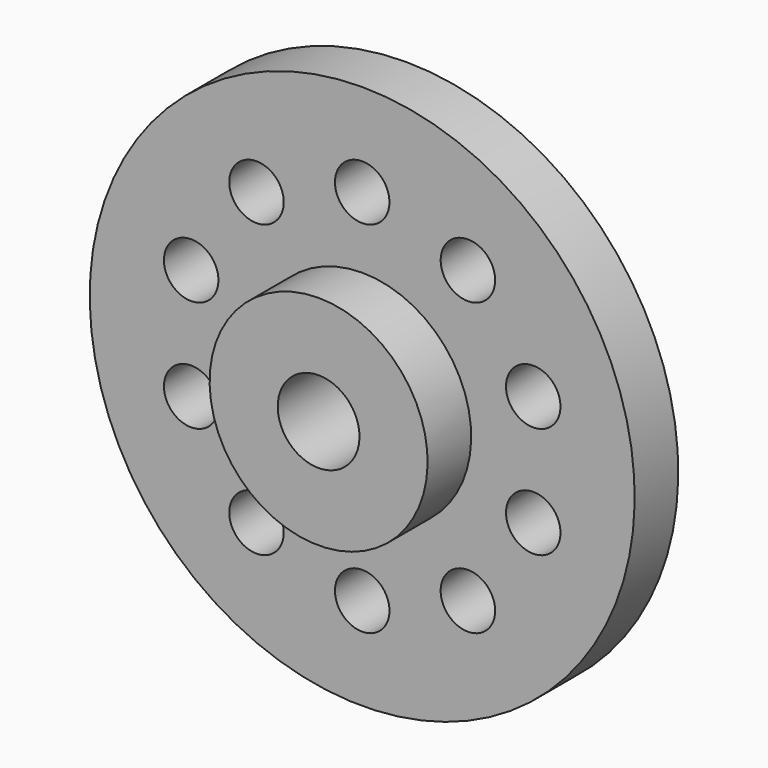
from build123d import *

# Parameters (mm, degrees)
F3_D            = 12.7
F3_COPIES_COUNT = 10


# Not quite as in the source:
# - a pattern or mirror of a feature is missing from the dataset's text; its kind, count and spacing are read off the source's solid


with BuildPart() as f1:
    # F0 (on Right) → F1 (revolve)
    with BuildSketch(Plane.YZ):
        Polygon((-25.4, 25.4), (-25.4, 9.525), (0, 9.525), (0, 63.5), (-12.7, 63.5), (-12.7, 25.4), align=None)
    revolve(axis=Axis((0, -12.7, 0), (0, -1, 0)))

    # F3 (through all)
    with Locations(Plane(origin=(0, 0, 0), x_dir=(1, 0, 0), z_dir=(0, 1, 0))):
        with Locations((0, -41.91)):
            f3 = Hole(F3_D / 2)

    # F3_copies: F3 ×10 about axis
    f3_copies_axis = Axis((0, 0, 0), (0, 1, 0))
    for i in range(1, F3_COPIES_COUNT):
        add(f3.rotate(f3_copies_axis, i * 360 / F3_COPIES_COUNT), mode=Mode.SUBTRACT)


solid = f1.part
